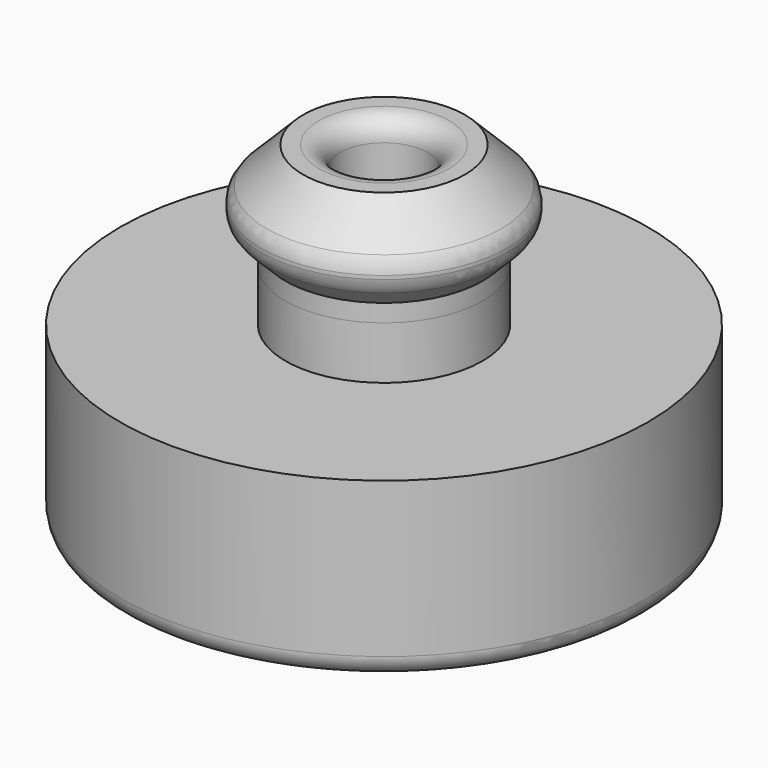
from build123d import *

# Parameters (mm, degrees)
F0_R        = 7.5
F1_DEPTH    = 5
F2_R        = 2.8
F3_DEPTH    = 1.5
F4_R        = 3.5
F5_DEPTH    = 3
F6_S5_R     = 2.8
F6_T6_DEPTH = 6
F7_R        = 1.25
F8_DEPTH    = 3.5
F9_R        = 0.6


# Not quite as in the source:
# - a fillet or chamfer that OpenCascade refuses, or shapes differently, is made with other operations: its cross-section is extruded or revolved along the edge and cut away or added
# - two fillets or chamfers of one size are made in one step


with BuildPart() as f1:
    # F0 (on Top) → F1 (new body)
    with BuildSketch(Plane.XY):
        Circle(F0_R)
    extrude(amount=F1_DEPTH)

    # F2 (on face) → F3 (join)
    with BuildSketch(Plane.XY.offset(5)):
        Circle(F2_R)
    extrude(amount=F3_DEPTH)

    # F4 (on face) → F5 (join)
    with BuildSketch(Plane.XY.offset(6.5)):
        Circle(F4_R)
    extrude(amount=F5_DEPTH)

    # F6: chamfer of 1.2 on 2 edges, made by hand


with BuildPart() as f6_tool2:
    # F6_s3 → F6_t4 (revolve)
    with BuildSketch(Plane.XZ):
        Polygon((3.5, 7.7), (2.3, 6.5), (3.5, 6.5), align=None)
    revolve(axis=Axis((0, 0, 6.5), (0, 0, 1)))

    # F6_s5 → F6_t6 (cut, symmetric)
    with BuildSketch(Plane.XY.offset(7.1)):
        Circle(F6_S5_R)
    extrude(amount=F6_T6_DEPTH, both=True, mode=Mode.SUBTRACT)


with BuildPart() as f1_1:
    add(f1.part)

    # F6_t1: cut F6_tool2
    add(f6_tool2.part, mode=Mode.SUBTRACT)

    # F6_s7 → F6_t8 (revolve, cut)
    with BuildSketch(Plane.XZ):
        Polygon((3.5, 8.3), (2.3, 9.5), (3.5, 9.5), align=None)
    revolve(axis=Axis((0, 0, 9.5), (0, 0, 1)), mode=Mode.SUBTRACT)

    # F7 (on face) → F8 (cut)
    with BuildSketch(Plane.XY.offset(9.5)):
        Circle(F7_R)
    extrude(amount=-F8_DEPTH, mode=Mode.SUBTRACT)

    # F9
    f9_edges = [f1_1.edges().sort_by_distance(p)[0] for p in [
        (-1.25, 0, 9.5),
        (-3.5, 0, 8.3),
        (-3.5, 0, 7.7),
        (-7.5, 0, 0),
    ]]
    fillet(f9_edges, radius=F9_R)


solid = f1_1.part
